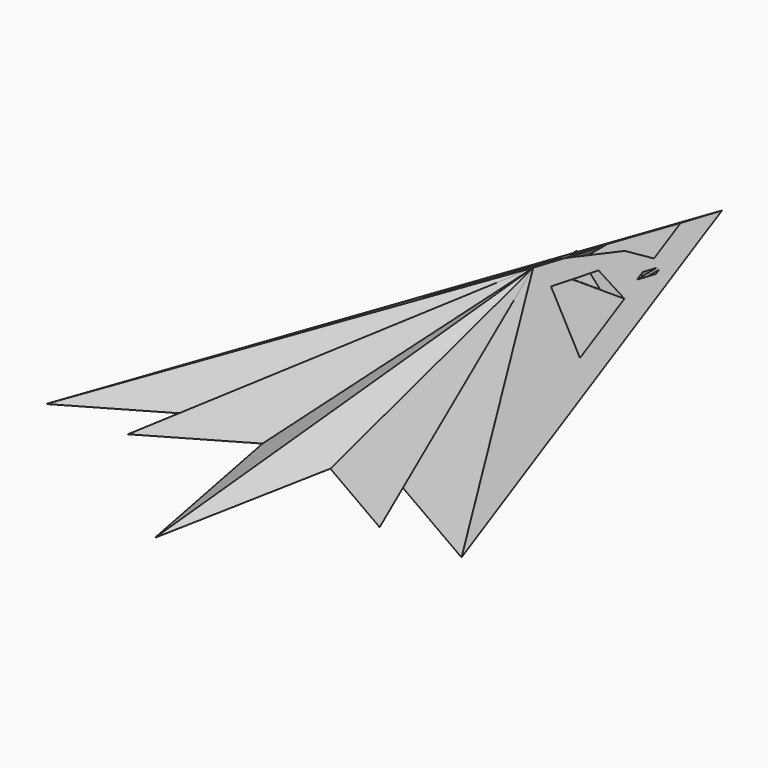
from build123d import *

# Parameters (mm, degrees)
F6_DEPTH  = 166.5272102769
F9_DEPTH  = 101.6
F10_DEPTH = 39.8337877091
F12_W     = 2.54
F12_H     = 2.54
F13_DEPTH = 25.4
F14_DEPTH = 12.7
F15_R     = 22.225
F16_DEPTH = 2.54


# Not quite as in the source:
# - the program builds the solid bodies; features that only make, move or delete a surface that nothing else refers to are left out


with BuildPart() as f3:
    # F0 (on Top) → F3 section 0
    with BuildSketch(Plane.XY, mode=Mode.PRIVATE) as f3_s0:
        Polygon((115.7262101769, -133.7715089321), (0, 192.2327876091), (-115.7262101769, -133.7715089321), (-38.9538705349, -89.2658084631), (-70.1078623533, -133.7715089321), (-18.8981407312, -104.0847162377), (0, -202.7553617954), (18.8981407312, -104.0847162377), (70.1078623533, -133.7715089321), (38.9538705349, -89.2658084631), align=None)
    loft([f3_s0.sketch, Vertex(0, 60.7637315989, 25.4)])

    # F5 (on offset) → F6 (cut, through all)
    with BuildSketch(Plane.YZ.offset(50.8)):
        Polygon((94.1726788878, 13.6528518051), (60.1693615317, 19.8352746665), (36.985270679, 5.446716453), (92.6806539106, 5.446716453), align=None)
    extrude(amount=-F6_DEPTH, mode=Mode.SUBTRACT)

    # F8 (on offset) → F9 (cut)
    with BuildSketch(Plane.XZ.offset(-152.4)):
        Polygon((-12.4854929745, 5.5678542703), (11.810598895, 5.5678542703), (4.7242408618, 11.641876772), (0, 21.0903566331), (-5.3991349414, 11.641876772), align=None)
    extrude(amount=F9_DEPTH, mode=Mode.SUBTRACT)

    # F10 (cut, through all): a face of the model
    f10_faces = [f3.faces().sort_by_distance(p)[0] for p in [
        (0, 152.4, 6.2771523841),
    ]]
    extrude(f10_faces, amount=-F10_DEPTH, mode=Mode.SUBTRACT)

    # F12 (on offset) → F13 (join)
    with BuildSketch(Plane.XZ.offset(-127)):
        with Locations((17.467392717, 4.4757343051)):
            Rectangle(F12_W, F12_H)
        with Locations((-17.467392717, 4.4757343051)):
            Rectangle(F12_W, F12_H)
    extrude(amount=F13_DEPTH)

    # F14 (cut): faces of the model
    f14_faces = [f3.faces().sort_by_distance(p)[0] for p in [
        (17.5136661011, 127, 4.5302328808),
        (-17.5136661011, 127, 4.5302328808),
    ]]
    extrude(f14_faces, amount=-F14_DEPTH, mode=Mode.SUBTRACT)

    # F15 (on face) → F16 (cut)
    with BuildSketch(Plane(origin=(0, 0, 0), x_dir=(1, 0, 0), z_dir=(0, 0, -1))):
        with Locations((-51.2486876787, 53.3265663744)):
            Circle(F15_R)
        with Locations((51.2486876787, 53.3265663744)):
            Circle(F15_R)
        with Locations((0, 0.0474439003)):
            Circle(F15_R)
        with Locations((0, -88.4402606044)):
            Circle(F15_R)
    extrude(amount=-F16_DEPTH, mode=Mode.SUBTRACT)


solid = f3.part
